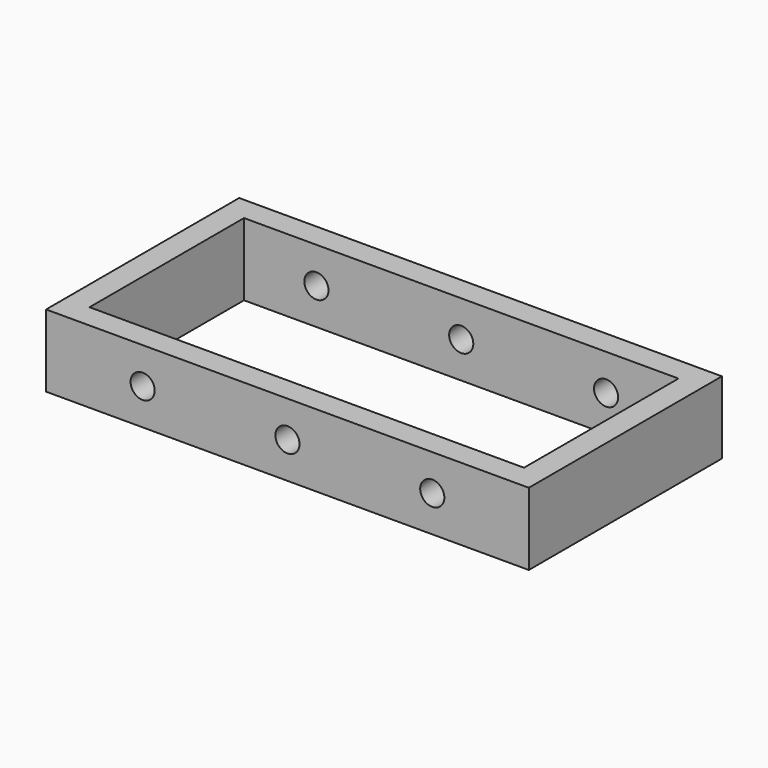
from build123d import *

# Parameters (mm, degrees)
F0_W     = 100
F0_H     = 50
F0_W_2   = 90
F0_H_2   = 40
F1_DEPTH = 7.5
F2_R     = 2.5
F3_DEPTH = 25


with BuildPart() as f1:
    # F0 (on Top) → F1 (new body, symmetric)
    with BuildSketch(Plane.XY):
        Rectangle(F0_W, F0_H)
        Rectangle(F0_W_2, F0_H_2, mode=Mode.SUBTRACT)
    extrude(amount=F1_DEPTH, both=True)

    # F2 (on Front) → F3 (cut, symmetric)
    with BuildSketch(Plane.XZ):
        Circle(F2_R)
        with Locations((-30, 0)):
            Circle(F2_R)
        with Locations((30, 0)):
            Circle(F2_R)
    extrude(amount=F3_DEPTH, both=True, mode=Mode.SUBTRACT)


solid = f1.part
